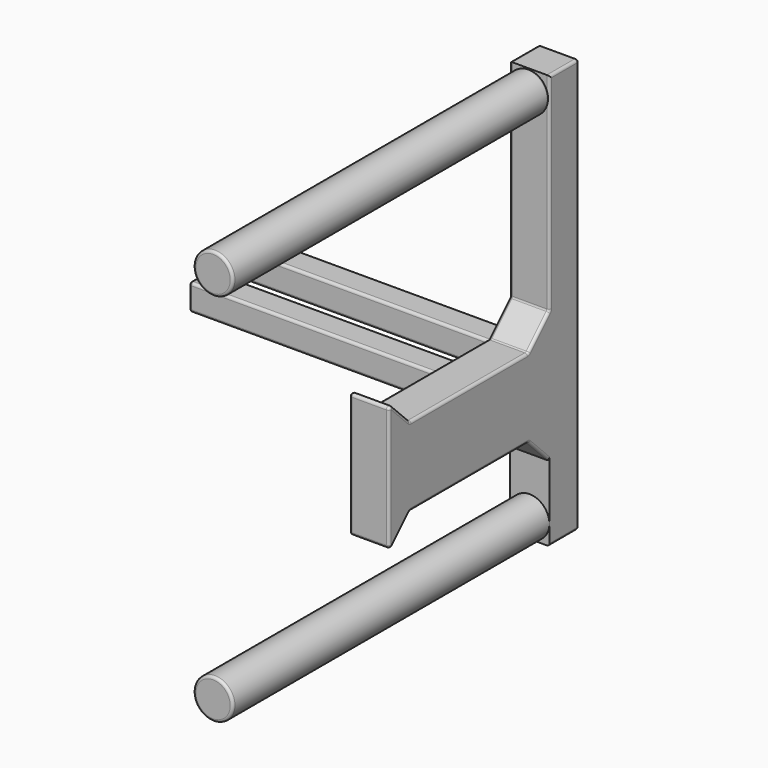
from build123d import *

# Parameters (mm, degrees)
F0_R      = 3.75
F1_DEPTH  = 75
F2_W      = 7.5
F2_H      = 78.5
F3_DEPTH  = 7
F4_W      = 7.5
F4_H      = 25
F5_DEPTH  = 45
F7_DEPTH  = 25
F8_W      = 18
F8_H      = 5
F9_DEPTH  = 52
F10_W     = 47
F10_H     = 8
F11_DEPTH = 25
F12_R     = 0.5
F12_2_R   = 0.5
F12_3_R   = 0.5


with BuildPart() as f1:
    # F0 (on Front) → F1 (new body)
    with BuildSketch(Plane.XZ):
        with Locations((0, 35.5)):
            Circle(F0_R)
    extrude(amount=F1_DEPTH)

    # F12
    f12_edges = [f1.edges().sort_by_distance(p)[0] for p in [
        (-3.75, -75, 35.5),
        (3.75, -37.5, 35.5),
        (-3.75, 0, 35.5),
    ]]
    fillet(f12_edges, radius=F12_R)


with BuildPart() as f1b:
    # F0 (on Front) → F1, piece 2 (new body)
    with BuildSketch(Plane.XZ):
        with Locations((0, -35.5)):
            Circle(F0_R)
    extrude(amount=F1_DEPTH)

    # F12#2
    f12_2_edges = [f1b.edges().sort_by_distance(p)[0] for p in [
        (-3.75, -75, -35.5),
    ]]
    fillet(f12_2_edges, radius=F12_2_R)


with BuildPart() as f3:
    # F2 (on Front) → F3 (new body)
    with BuildSketch(Plane.XZ):
        Rectangle(F2_W, F2_H)
    extrude(amount=-F3_DEPTH)

    # F4 (on face) → F5 (join)
    with BuildSketch(Plane(origin=(0, 7, 0), x_dir=(-1, 0, 0), z_dir=(0, 1, 0))):
        with Locations((0, -12.5)):
            Rectangle(F4_W, F4_H)
    extrude(amount=-F5_DEPTH)

    # F6 (on face) → F7 (cut)
    with BuildSketch(Plane.YZ.offset(3.75)):
        Polygon((0, 0), (-38, 0), (-33, -5), (-5, -5), align=None)
        Polygon((-33, -20), (-38, -25), (0, -25), (-5, -20), align=None)
    extrude(amount=-F7_DEPTH, mode=Mode.SUBTRACT)

    # F8 (on face) → F9 (join)
    with BuildSketch(Plane(origin=(-3.75, 0, 0), x_dir=(0, -1, 0), z_dir=(-1, 0, 0))):
        with Locations((2, -12.5)):
            Rectangle(F8_W, F8_H)
    extrude(amount=F9_DEPTH)

    # F10 (on face) → F11 (cut)
    with BuildSketch(Plane.XY.offset(-10)):
        with Locations((-32.25, -2)):
            Rectangle(F10_W, F10_H)
    extrude(amount=-F11_DEPTH, mode=Mode.SUBTRACT)

    # F12#3
    f12_3_edges = [f3.edges().sort_by_distance(p)[0] for p in [
        (-55.75, 2, -12.5),
        (-55.75, -6, -12.5),
        (-8.75, 2, -12.5),
        (-3.75, 3.5, -39.25),
        (0, 7, -39.25),
        (3.75, 3.5, -39.25),
        (-3.75, 7, -27.125),
        (3.75, 7, 0),
        (-29.75, 7, -15),
        (-29.75, 7, -10),
        (-3.75, 7, 14.625),
        (3.75, -19, -20),
        (3.75, -2.5, -22.5),
        (-3.75, -2.5, -22.5),
        (-3.75, -19, -20),
        (0, -5, -20),
        (0, 0, 0),
        (0, -5, -5),
        (3.75, -2.5, -2.5),
        (3.75, -19, -5),
        (-3.75, -2.5, -2.5),
        (-3.75, 0, 19.625),
        (-3.75, -35.5, -2.5),
        (-29.75, -11, -15),
        (-29.75, -11, -10),
        (-3.75, -11, -12.5),
        (-55.75, -11, -12.5),
        (0, 7, 39.25),
        (3.75, 3.5, 39.25),
        (-3.75, 3.5, 39.25),
        (0, -38, -25),
        (0, -38, 0),
        (3.75, -38, -12.5),
        (-3.75, -38, -12.5),
        (3.75, -35.5, -22.5),
        (-3.75, -35.5, -22.5),
        (0, -33, -20),
        (3.75, -35.5, -2.5),
        (0, -33, -5),
        (-55.75, 4.5, -15),
        (-55.75, 7, -12.5),
        (-55.75, 4.5, -10),
        (-55.75, -8.5, -15),
        (-55.75, -8.5, -10),
        (-32.25, -6, -10),
        (-8.75, -6, -12.5),
        (-32.25, -6, -15),
        (3.75, 0, 19.625),
        (-3.75, -19, -5),
        (-3.75, -2, -15),
        (-3.75, -2, -10),
        (-32.25, 2, -10),
        (-8.75, -2, -10),
        (-8.75, -2, -15),
        (-32.25, 2, -15),
    ]]
    fillet(f12_3_edges, radius=F12_3_R)


solid = Compound([f1.part, f1b.part, f3.part])
